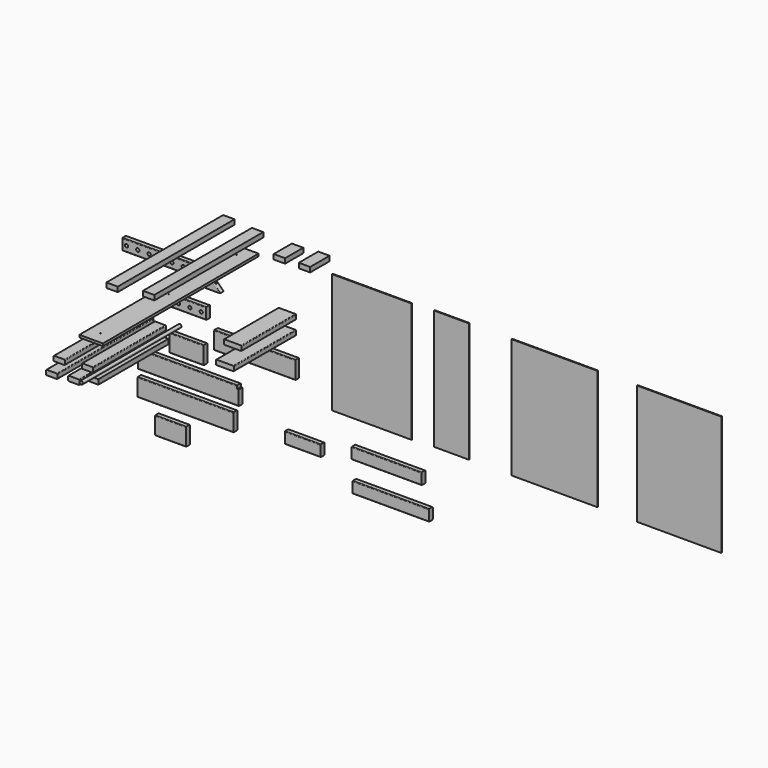
from build123d import *

# Parameters (mm, degrees)
F0_W      = 88.9
F0_H      = 38.1
F1_DEPTH  = 939.8
F2_R      = 5.08
F3_DEPTH  = 863.6
F4_DEPTH  = 711.2
F0_W_2    = 266.7
F0_H_2    = 139.7
F5_DEPTH  = 38.1
F6_DEPTH  = 38.1
F7_R      = 5.08
F7_2_R    = 5.08
F7_3_R    = 5.08
F7_4_R    = 5.08
F8_DEPTH  = 723.9
F9_R      = 5.08
F10_DEPTH = 196.85
F11_DEPTH = 685.8
F12_DEPTH = 571.5
F0_R      = 12.7
F13_DEPTH = 965.2
F14_DEPTH = 38.1
F16_DEPTH = 38.1
F17_R     = 5.08
F17_2_R   = 5.08
F0_W_3    = 749.3
F18_DEPTH = 38.1
F19_R     = 5.08
F0_W_4    = 622.3
F0_H_3    = 939.8
F20_DEPTH = 6.35
F0_W_5    = 273.05
F21_DEPTH = 6.35
F0_W_6    = 673.1
F22_DEPTH = 6.35
F23_DEPTH = 38.1
F24_R     = 5.08
F26_START = -38.1
F26_DEPTH = 38.1
F28_START = -25.4
F28_DEPTH = 50.8
F0_W_7    = 139.7
F29_DEPTH = 533.4
F30_DEPTH = 609.6
F31_R     = 5.08
F31_2_R   = 5.08
F0_W_8    = 635
F32_DEPTH = 38.1
F33_R     = 5.08
F0_W_9    = 546.1
F0_H_4    = 88.9
F34_DEPTH = 38.1
F0_W_10   = 596.9
F35_DEPTH = 38.1
F36_R     = 5.08
F36_2_R   = 5.08
F0_W_11   = 279.4
F37_DEPTH = 38.1
F38_R     = 5.08
F0_W_12   = 241.3
F39_DEPTH = 38.1
F40_R     = 5.08
F0_W_13   = 660.4
F41_DEPTH = 6.35
F42_DEPTH = 1143
F43_DEPTH = 1066.8
F44_DEPTH = 177.8
F45_DEPTH = 190.5
F0_W_14   = 184.15
F0_H_5    = 19.05
F46_DEPTH = 1524
F47_R     = 3.175
F48_DEPTH = 50.8


# Not quite as in the source:
# - a feature names something its author has since deleted; it is built from what else it names


with BuildPart() as f1:
    # F0 (on Front) → F1 (new body)
    with BuildSketch(Plane.XZ):
        with Locations((-41.2130072497, 42.3422695577)):
            Rectangle(F0_W, F0_H)
    extrude(amount=F1_DEPTH)

    # F2
    f2_edges = [f1.edges().sort_by_distance(p)[0] for p in [
        (-85.663007, -469.9, 61.39227),
        (-85.663007, -469.9, 23.29227),
        (3.236993, -469.9, 61.39227),
        (3.236993, -469.9, 23.29227),
    ]]
    fillet(f2_edges, radius=F2_R)


with BuildPart() as f3:
    # F0 (on Front) → F3 (new body)
    with BuildSketch(Plane.XZ):
        with Locations((-42.9722144485, 107.2543614984)):
            Rectangle(F0_W, F0_H)
    extrude(amount=F3_DEPTH)

    # F7
    f7_edges = [f3.edges().sort_by_distance(p)[0] for p in [
        (1.477786, -431.8, 126.304361),
        (1.477786, -431.8, 88.204361),
        (-87.422214, -431.8, 88.204361),
        (-87.422214, -431.8, 126.304361),
    ]]
    fillet(f7_edges, radius=F7_R)


with BuildPart() as f4:
    # F0 (on Front) → F4 (new body)
    with BuildSketch(Plane.XZ):
        with Locations((56.0904666066, 25.0534138151)):
            Rectangle(F0_W, F0_H)
    extrude(amount=F4_DEPTH)

    # F7#2
    f7_2_edges = [f4.edges().sort_by_distance(p)[0] for p in [
        (100.540467, -355.6, 44.103414),
        (100.540467, -355.6, 6.003414),
        (11.640467, -355.6, 6.003414),
        (11.640467, -355.6, 44.103414),
    ]]
    fillet(f7_2_edges, radius=F7_2_R)


with BuildPart() as f5:
    # F0 (on Front) → F5 (new body)
    with BuildSketch(Plane.XZ):
        with Locations((292.5869745441, -41.1412539788)):
            Rectangle(F0_W_2, F0_H_2)
    extrude(amount=F5_DEPTH)

    # F7#4
    f7_4_edges = [f5.edges().sort_by_distance(p)[0] for p in [
        (292.586975, -38.1, 28.708746),
        (292.586975, 0, 28.708746),
        (292.586975, -38.1, -110.991254),
        (292.586975, 0, -110.991254),
    ]]
    fillet(f7_4_edges, radius=F7_4_R)


with BuildPart() as f6:
    # F0 (on Front) → F6 (new body)
    with BuildSketch(Plane.XZ):
        Polygon((-86.6090655327, -163.0578890324), (-86.6090655327, -302.7578890324), (700.7909344673, -302.7578890324), (700.7909344673, -188.4578890324), (688.0909344673, -188.4578890324), (688.0909344673, -163.0578890324), align=None)
    extrude(amount=F6_DEPTH)

    # F7#3
    f7_3_edges = [f6.edges().sort_by_distance(p)[0] for p in [
        (300.740934, -38.1, -163.057889),
        (300.740934, 0, -163.057889),
        (307.090934, -38.1, -302.757889),
        (307.090934, 0, -302.757889),
    ]]
    fillet(f7_3_edges, radius=F7_3_R)


with BuildPart() as f8:
    # F0 (on Front) → F8 (new body)
    with BuildSketch(Plane.XZ):
        with Locations((-41.1397143483, -86.2058347583)):
            Rectangle(F0_W, F0_H)
    extrude(amount=F8_DEPTH)

    # F9
    f9_edges = [f8.edges().sort_by_distance(p)[0] for p in [
        (3.310286, -361.95, -67.155835),
        (-85.589714, -361.95, -67.155835),
        (3.310286, -361.95, -105.255835),
        (-85.589714, -361.95, -105.255835),
    ]]
    fillet(f9_edges, radius=F9_R)


with BuildPart() as f10:
    # F0 (on Front) → F10 (new body)
    with BuildSketch(Plane.XZ):
        with Locations((-41.2697750859, -22.8207504869)):
            Rectangle(F0_W, F0_H)
    extrude(amount=F10_DEPTH)


with BuildPart() as f11:
    # F0 (on Front) → F11 (new body)
    with BuildSketch(Plane.XZ):
        with Locations((76.0908796668, -60.551585865)):
            Rectangle(F0_W, F0_H)
    extrude(amount=F11_DEPTH)


with BuildPart() as f12:
    # F0 (on Front) → F12 (new body)
    with BuildSketch(Plane.XZ):
        with Locations((222.5183992863, 113.1555864096)):
            Rectangle(F0_W, F0_H)
    extrude(amount=F12_DEPTH)


with BuildPart() as f13:
    # F0 (on Front) → F13 (new body)
    with BuildSketch(Plane.XZ):
        with Locations((210.0020796061, 76.8552199006)):
            Circle(F0_R)
    extrude(amount=F13_DEPTH)


with BuildPart() as f14:
    # F0 (on Front) → F14 (new body)
    with BuildSketch(Plane.XZ):
        Polygon((445.7719624043, 297.4565924644), (13.9719624043, 297.4565924644), (13.9719624043, 253.0065924644), (13.9719624043, 208.5565924644), (445.7719624043, 208.5565924644), align=None)
        with BuildLine():
            ThreePointArc((64.7719624043, 253.0065924644), (52.0719624043, 240.3065924644), (39.3719624043, 253.0065924644))
            ThreePointArc((39.3719624043, 253.0065924644), (52.0719624043, 265.7065924644), (64.7719624043, 253.0065924644))
        make_face(mode=Mode.SUBTRACT)
        with BuildLine():
            ThreePointArc((153.6719624043, 253.0065924644), (140.9719624043, 240.3065924644), (128.2719624043, 253.0065924644))
            ThreePointArc((128.2719624043, 253.0065924644), (140.9719624043, 265.7065924644), (153.6719624043, 253.0065924644))
        make_face(mode=Mode.SUBTRACT)
        with BuildLine():
            ThreePointArc((242.5719624043, 253.0065924644), (229.8719624043, 240.3065924644), (217.1719624043, 253.0065924644))
            ThreePointArc((217.1719624043, 253.0065924644), (229.8719624043, 265.7065924644), (242.5719624043, 253.0065924644))
        make_face(mode=Mode.SUBTRACT)
        with BuildLine():
            ThreePointArc((331.4719624043, 253.0065924644), (318.7719624043, 240.3065924644), (306.0719624043, 253.0065924644))
            ThreePointArc((306.0719624043, 253.0065924644), (318.7719624043, 265.7065924644), (331.4719624043, 253.0065924644))
        make_face(mode=Mode.SUBTRACT)
        with BuildLine():
            ThreePointArc((420.3719624043, 253.0065924644), (407.6719624043, 240.3065924644), (394.9719624043, 253.0065924644))
            ThreePointArc((394.9719624043, 253.0065924644), (407.6719624043, 265.7065924644), (420.3719624043, 253.0065924644))
        make_face(mode=Mode.SUBTRACT)
    extrude(amount=F14_DEPTH)

    # F17#2
    f17_2_edges = [f14.edges().sort_by_distance(p)[0] for p in [
        (229.871962, -38.1, 297.456592),
        (229.871962, -38.1, 208.556592),
        (229.871962, 0, 208.556592),
        (229.871962, 0, 297.456592),
    ]]
    fillet(f17_2_edges, radius=F17_2_R)


with BuildPart() as f16:
    # F0 (on Front) → F16 (new body)
    with BuildSketch(Plane.XZ):
        Polygon((387.35, 562.6177789211), (-209.55, 562.6177789211), (-209.55, 518.1677789211), (-209.55, 473.7177789211), (387.35, 473.7177789211), align=None)
        with BuildLine():
            ThreePointArc((-165.1, 518.1677789211), (-177.8, 505.4677789211), (-190.5, 518.1677789211))
            ThreePointArc((-190.5, 518.1677789211), (-177.8, 530.8677789211), (-165.1, 518.1677789211))
        make_face(mode=Mode.SUBTRACT)
        with BuildLine():
            ThreePointArc((-76.2, 518.1677789211), (-88.9, 505.4677789211), (-101.6, 518.1677789211))
            ThreePointArc((-101.6, 518.1677789211), (-88.9, 530.8677789211), (-76.2, 518.1677789211))
        make_face(mode=Mode.SUBTRACT)
        with BuildLine():
            ThreePointArc((12.7, 518.1677789211), (0, 505.4677789211), (-12.7, 518.1677789211))
            ThreePointArc((-12.7, 518.1677789211), (0, 530.8677789211), (12.7, 518.1677789211))
        make_face(mode=Mode.SUBTRACT)
        with BuildLine():
            ThreePointArc((101.6, 518.1677789211), (88.9, 505.4677789211), (76.2, 518.1677789211))
            ThreePointArc((76.2, 518.1677789211), (88.9, 530.8677789211), (101.6, 518.1677789211))
        make_face(mode=Mode.SUBTRACT)
        with BuildLine():
            ThreePointArc((190.5, 518.1677789211), (177.8, 505.4677789211), (165.1, 518.1677789211))
            ThreePointArc((165.1, 518.1677789211), (177.8, 530.8677789211), (190.5, 518.1677789211))
        make_face(mode=Mode.SUBTRACT)
        with BuildLine():
            ThreePointArc((279.4, 518.1677789211), (266.7, 505.4677789211), (254, 518.1677789211))
            ThreePointArc((254, 518.1677789211), (266.7, 530.8677789211), (279.4, 518.1677789211))
        make_face(mode=Mode.SUBTRACT)
        with BuildLine():
            ThreePointArc((368.3, 518.1677789211), (355.6, 505.4677789211), (342.9, 518.1677789211))
            ThreePointArc((342.9, 518.1677789211), (355.6, 530.8677789211), (368.3, 518.1677789211))
        make_face(mode=Mode.SUBTRACT)
    extrude(amount=F16_DEPTH)

    # F17
    f17_edges = [f16.edges().sort_by_distance(p)[0] for p in [
        (88.9, -38.1, 562.617779),
        (88.9, -38.1, 473.717779),
        (88.9, 0, 473.717779),
        (88.9, 0, 562.617779),
    ]]
    fillet(f17_edges, radius=F17_R)


with BuildPart() as f18:
    # F0 (on Front) → F18 (new body)
    with BuildSketch(Plane.XZ):
        with Locations((285.0359097481, -427.6944674492)):
            Rectangle(F0_W_3, F0_H_2)
    extrude(amount=F18_DEPTH)

    # F19
    f19_edges = [f18.edges().sort_by_distance(p)[0] for p in [
        (285.03591, -38.1, -357.844467),
        (285.03591, -38.1, -497.544467),
        (285.03591, 0, -357.844467),
        (285.03591, 0, -497.544467),
    ]]
    fillet(f19_edges, radius=F19_R)


with BuildPart() as f20:
    # F0 (on Front) → F20 (new body)
    with BuildSketch(Plane.XZ):
        with Locations((1718.5346885681, 355.0495459676)):
            Rectangle(F0_W_4, F0_H_3)
    extrude(amount=F20_DEPTH)


with BuildPart() as f21:
    # F0 (on Front) → F21 (new body)
    with BuildSketch(Plane.XZ):
        with Locations((2340.9749938965, 363.9606936812)):
            Rectangle(F0_W_5, F0_H_3)
    extrude(amount=F21_DEPTH)


with BuildPart() as f22:
    # F0 (on Front) → F22 (new body)
    with BuildSketch(Plane.XZ):
        with Locations((3148.1723812103, 363.9606936812)):
            Rectangle(F0_W_6, F0_H_3)
    extrude(amount=F22_DEPTH)


with BuildPart() as f23:
    # F0 (on Front) → F23 (new body)
    with BuildSketch(Plane.XZ):
        Polygon((555.9982657433, 428.1938076019), (416.2982657433, 567.8938076019), (416.2982657433, 428.1938076019), align=None)
    extrude(amount=F23_DEPTH)

    # F24
    f24_edges = [f23.edges().sort_by_distance(p)[0] for p in [
        (486.148266, -38.1, 498.043808),
        (486.148266, 0, 498.043808),
    ]]
    fillet(f24_edges, radius=F24_R)

    # F25 (on face) → F26 (cut)
    with BuildSketch(Plane(origin=(0, 0, 428.1938076019), x_dir=(1, 0, 0), z_dir=(0, 0, -1)).offset(F26_START)):
        with BuildLine():
            ThreePointArc((511.5482657433, 19.05), (505.1982657433, 25.4), (498.8482657433, 19.05))
            ThreePointArc((498.8482657433, 19.05), (505.1982657433, 12.7), (511.5482657433, 19.05))
        make_face()
    extrude(amount=-F26_DEPTH, mode=Mode.SUBTRACT)

    # F27 (on face) → F28 (cut)
    with BuildSketch(Plane(origin=(416.2982657433, 0, 0), x_dir=(0, -1, 0), z_dir=(-1, 0, 0)).offset(F28_START)):
        with BuildLine():
            ThreePointArc((25.4, 517.0938076019), (14.5598719395, 521.5839356625), (19.05, 510.7438076019))
            ThreePointArc((19.05, 510.7438076019), (23.5401280605, 512.6036795414), (25.4, 517.0938076019))
        make_face()
    extrude(amount=-F28_DEPTH, mode=Mode.SUBTRACT)


with BuildPart() as f29:
    # F0 (on Front) → F29 (new body)
    with BuildSketch(Plane.XZ):
        with Locations((1050.7598794937, 434.0879002094)):
            Rectangle(F0_W_7, F0_H)
    extrude(amount=F29_DEPTH)

    # F31
    f31_edges = [f29.edges().sort_by_distance(p)[0] for p in [
        (980.909879, -266.7, 453.1379),
        (980.909879, -266.7, 415.0379),
        (1120.609879, -266.7, 415.0379),
        (1120.609879, -266.7, 453.1379),
    ]]
    fillet(f31_edges, radius=F31_R)


with BuildPart() as f30:
    # F0 (on Front) → F30 (new body)
    with BuildSketch(Plane.XZ):
        with Locations((1050.7598794937, 324.8656967163)):
            Rectangle(F0_W_7, F0_H)
    extrude(amount=F30_DEPTH)

    # F31#2
    f31_2_edges = [f30.edges().sort_by_distance(p)[0] for p in [
        (980.909879, -304.8, 343.915697),
        (980.909879, -304.8, 305.815697),
        (1120.609879, -304.8, 305.815697),
        (1120.609879, -304.8, 343.915697),
    ]]
    fillet(f31_2_edges, radius=F31_2_R)


with BuildPart() as f32:
    # F0 (on Front) → F32 (new body)
    with BuildSketch(Plane.XZ):
        with Locations((826.8567239761, 90.9486305028)):
            Rectangle(F0_W_8, F0_H_2)
    extrude(amount=F32_DEPTH)

    # F33
    f33_edges = [f32.edges().sort_by_distance(p)[0] for p in [
        (826.856724, -38.1, 21.098631),
        (826.856724, -38.1, 160.798631),
        (826.856724, 0, 160.798631),
        (826.856724, 0, 21.098631),
    ]]
    fillet(f33_edges, radius=F33_R)


with BuildPart() as f34:
    # F0 (on Front) → F34 (new body)
    with BuildSketch(Plane.XZ):
        with Locations((1859.3762414932, -337.8479032993)):
            Rectangle(F0_W_9, F0_H_4)
    extrude(amount=F34_DEPTH)

    # F36
    f36_edges = [f34.edges().sort_by_distance(p)[0] for p in [
        (1859.376241, -38.1, -293.397903),
        (1859.376241, -38.1, -382.297903),
        (1859.376241, 0, -293.397903),
        (1859.376241, 0, -382.297903),
    ]]
    fillet(f36_edges, radius=F36_R)


with BuildPart() as f35:
    # F0 (on Front) → F35 (new body)
    with BuildSketch(Plane.XZ):
        with Locations((1892.1740123749, -570.966765213)):
            Rectangle(F0_W_10, F0_H_4)
    extrude(amount=F35_DEPTH)

    # F36#2
    f36_2_edges = [f35.edges().sort_by_distance(p)[0] for p in [
        (1892.174012, -38.1, -526.516765),
        (1892.174012, -38.1, -615.416765),
        (1892.174012, 0, -526.516765),
        (1892.174012, 0, -615.416765),
    ]]
    fillet(f36_2_edges, radius=F36_2_R)


with BuildPart() as f37:
    # F0 (on Front) → F37 (new body)
    with BuildSketch(Plane.XZ):
        with Locations((1202.080424118, -401.7872362614)):
            Rectangle(F0_W_11, F0_H_4)
    extrude(amount=F37_DEPTH)

    # F38
    f38_edges = [f37.edges().sort_by_distance(p)[0] for p in [
        (1202.080424, -38.1, -446.237236),
        (1202.080424, 0, -446.237236),
        (1202.080424, 0, -357.337236),
        (1202.080424, -38.1, -357.337236),
    ]]
    fillet(f38_edges, radius=F38_R)


with BuildPart() as f39:
    # F0 (on Front) → F39 (new body)
    with BuildSketch(Plane.XZ):
        with Locations((167.695515728, -647.5772537231)):
            Rectangle(F0_W_12, F0_H_2)
    extrude(amount=F39_DEPTH)

    # F40
    f40_edges = [f39.edges().sort_by_distance(p)[0] for p in [
        (167.695516, -38.1, -577.727254),
        (167.695516, -38.1, -717.427254),
        (167.695516, 0, -717.427254),
        (167.695516, 0, -577.727254),
    ]]
    fillet(f40_edges, radius=F40_R)


with BuildPart() as f41:
    # F0 (on Front) → F41 (new body)
    with BuildSketch(Plane.XZ):
        with Locations((4124.585433197, 363.9606936812)):
            Rectangle(F0_W_13, F0_H_3)
    extrude(amount=F41_DEPTH)


with BuildPart() as f42:
    # F0 (on Front) → F42 (new body)
    with BuildSketch(Plane.XZ):
        with Locations((593.6150997162, 931.8633058548)):
            Rectangle(F0_W, F0_H)
    extrude(amount=F42_DEPTH)


with BuildPart() as f43:
    # F0 (on Front) → F43 (new body)
    with BuildSketch(Plane.XZ):
        with Locations((818.6690061569, 916.6569688797)):
            Rectangle(F0_W, F0_H)
    extrude(amount=F43_DEPTH)


with BuildPart() as f44:
    # F0 (on Front) → F44 (new body)
    with BuildSketch(Plane.XZ):
        with Locations((1131.9196670532, 910.5744340897)):
            Rectangle(F0_W, F0_H)
    extrude(amount=F44_DEPTH)


with BuildPart() as f45:
    # F0 (on Front) → F45 (new body)
    with BuildSketch(Plane.XZ):
        with Locations((1338.0954711914, 922.3245957375)):
            Rectangle(F0_W, F0_H)
    extrude(amount=F45_DEPTH)


with BuildPart() as f46:
    # F0 (on Front) → F46 (new body)
    with BuildSketch(Plane.XZ):
        with Locations((734.4905786514, 765.8224691391)):
            Rectangle(F0_W_14, F0_H_5)
    extrude(amount=F46_DEPTH)

    # F47 (on face) → F48 (cut)
    with BuildSketch(Plane(origin=(0, 0, 756.2974691391), x_dir=(1, 0, 0), z_dir=(0, 0, -1))):
        with BuildLine():
            ThreePointArc((734.4905786514, 95.25), (729.0705146212, 97.4950640303), (731.3155786514, 92.075))
            Line((731.3155786514, 92.075), (731.3155786514, 95.25))
            Line((731.3155786514, 95.25), (734.4905786514, 95.25))
        make_face()
        with BuildLine():
            Line((731.3155786514, 95.25), (731.3155786514, 92.075))
            ThreePointArc((731.3155786514, 92.075), (733.5606426817, 93.0049359697), (734.4905786514, 95.25))
            Line((734.4905786514, 95.25), (731.3155786514, 95.25))
        make_face()
        with Locations((731.3155786514, 762)):
            Circle(F47_R)
        with BuildLine():
            ThreePointArc((731.3155786514, 1431.925), (729.0705146212, 1426.5049359697), (734.4905786514, 1428.75))
            Line((734.4905786514, 1428.75), (731.3155786514, 1428.75))
            Line((731.3155786514, 1428.75), (731.3155786514, 1431.925))
        make_face()
        with BuildLine():
            Line((731.3155786514, 1428.75), (734.4905786514, 1428.75))
            ThreePointArc((734.4905786514, 1428.75), (733.5606426817, 1430.9950640303), (731.3155786514, 1431.925))
            Line((731.3155786514, 1431.925), (731.3155786514, 1428.75))
        make_face()
    extrude(amount=-F48_DEPTH, mode=Mode.SUBTRACT)


solid = Compound([f1.part, f3.part, f4.part, f5.part, f6.part, f8.part, f10.part, f11.part, f13.part, f14.part, f16.part, f18.part, f20.part, f21.part, f22.part, f23.part, f29.part, f30.part, f32.part, f34.part, f35.part, f37.part, f39.part, f41.part, f42.part, f43.part, f44.part, f45.part, f46.part])
